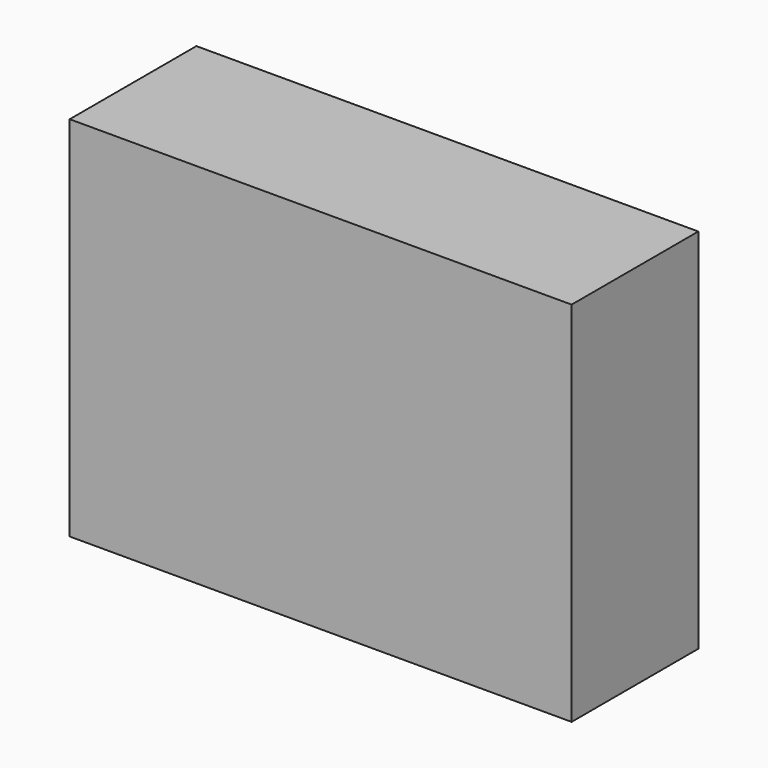
from build123d import *

# Parameters (mm, degrees)
F0_W     = 80.4933309555
F0_H     = 58.917850256
F1_DEPTH = 25.4


# Not quite as in the source:
# - the program builds the solid bodies; features that only make, move or delete a surface that nothing else refers to are left out


with BuildPart() as f1:
    # F0 (on Front) → F1 (new body)
    with BuildSketch(Plane.XZ):
        Rectangle(F0_W, F0_H)
    extrude(amount=F1_DEPTH)


solid = f1.part
